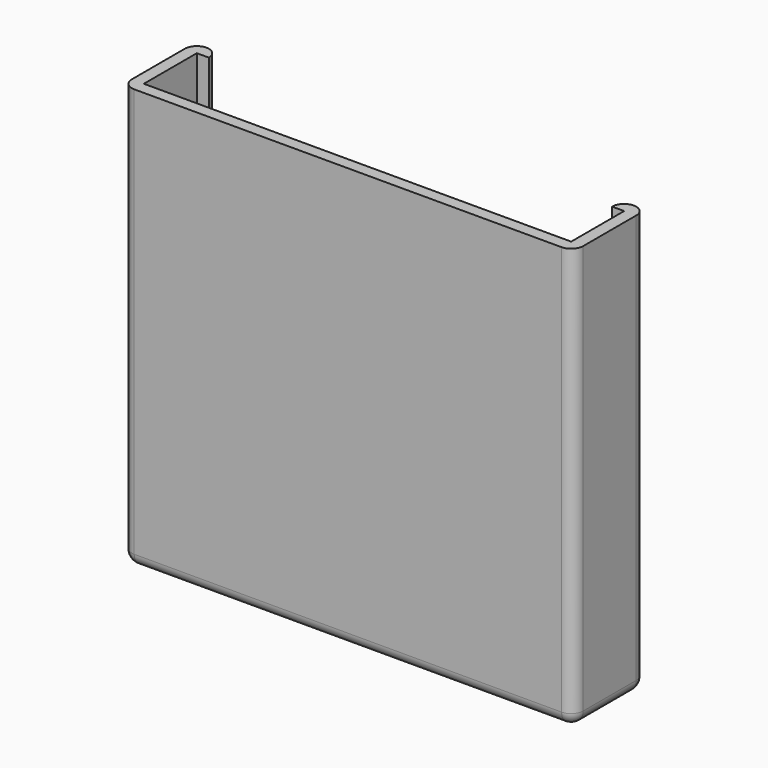
from build123d import *

# Parameters (mm, degrees)
F0_DEPTH     = 70
F1_W         = 75
F1_H         = 15
F4_DEPTH     = 2
F2_T1_DEPTH  = 11
F2_T3_DEPTH  = 73
F2_T5_DEPTH  = 67
F2_T7_DEPTH  = 71
F2_S11_W     = 2.04
F2_S11_H     = 2.04
F2_T12_DEPTH = 2.04
F2_S17_W     = 2.04
F2_S17_H     = 2.04
F2_T18_DEPTH = 2.04
F2_S23_W     = 2.04
F2_S23_H     = 2.04
F2_T24_DEPTH = 2.04
F2_S29_W     = 2.04
F2_S29_H     = 2.04
F2_T30_DEPTH = 2.04
F2_T37_DEPTH = 73
F2_T42_DEPTH = 72
F2_T50_DEPTH = 72
F2_T55_DEPTH = 73
F2_T62_DEPTH = 16
F2_T67_DEPTH = 16


# Not quite as in the source:
# - a fillet or chamfer that OpenCascade refuses, or shapes differently, is made with other operations: its cross-section is extruded or revolved along the edge and cut away or added
# - a feature names something its author has since deleted; it is built from what else it names


with BuildPart() as f0:
    # F3 (on Top) → F0 (new body)
    with BuildSketch(Plane.XY):
        Polygon((-37.5, 15), (-37.5, 0), (37.5, 0), (37.5, 15), (33.5, 15), (33.5, 13), (35.5, 13), (35.5, 2), (-35.5, 2), (-35.5, 13), (-33.5, 13), (-33.5, 15), align=None)
    extrude(amount=F0_DEPTH)

    # F1 (on face) → F4 (join)
    with BuildSketch(Plane(origin=(0, 0, 0), x_dir=(1, 0, 0), z_dir=(0, 0, -1))):
        with Locations((0, -7.5)):
            Rectangle(F1_W, F1_H)
    extrude(amount=-F4_DEPTH)

    # F2: fillet of radius 2 on 13 edges, made by hand

    # F2_s2 → F2_t1 (cut)
    with BuildSketch(Plane.XZ.offset(-13)):
        with BuildLine():
            ThreePointArc((37.5, 2), (36.9142135624, 0.5857864376), (35.5, 0))
            Line((35.5, 0), (37.5, 0))
            Line((37.5, 0), (37.5, 2))
        make_face()
        with BuildLine():
            ThreePointArc((-37.5, 2), (-36.9142135624, 0.5857864376), (-35.5, 0))
            Line((-35.5, 0), (-37.5, 0))
            Line((-37.5, 0), (-37.5, 2))
        make_face()
    extrude(amount=F2_T1_DEPTH, mode=Mode.SUBTRACT)

    # F2_s4 → F2_t3 (cut)
    with BuildSketch(Plane.XY.offset(2)):
        with BuildLine():
            ThreePointArc((-37.5, 2), (-36.9142135624, 0.5857864376), (-35.5, 0))
            Line((-35.5, 0), (-37.5, 0))
            Line((-37.5, 0), (-37.5, 2))
        make_face()
        with BuildLine():
            ThreePointArc((35.5, 0), (36.9142135624, 0.5857864376), (37.5, 2))
            Line((37.5, 2), (37.5, 0))
            Line((37.5, 0), (35.5, 0))
        make_face()
        with BuildLine():
            ThreePointArc((-37.5, 13), (-36.9142135624, 14.4142135624), (-35.5, 15))
            Line((-35.5, 15), (-37.5, 15))
            Line((-37.5, 15), (-37.5, 13))
        make_face()
        with BuildLine():
            ThreePointArc((37.5, 13), (36.9142135624, 14.4142135624), (35.5, 15))
            Line((35.5, 15), (37.5, 15))
            Line((37.5, 15), (37.5, 13))
        make_face()
        with BuildLine():
            ThreePointArc((-33.5, 13), (-34.0857864376, 14.4142135624), (-35.5, 15))
            Line((-35.5, 15), (-33.5, 15))
            Line((-33.5, 15), (-33.5, 13))
        make_face()
        with BuildLine():
            ThreePointArc((33.5, 13), (34.0857864376, 14.4142135624), (35.5, 15))
            Line((35.5, 15), (33.5, 15))
            Line((33.5, 15), (33.5, 13))
        make_face()
    extrude(amount=F2_T3_DEPTH, mode=Mode.SUBTRACT)

    # F2_s6 → F2_t5 (cut)
    with BuildSketch(Plane.YZ.offset(-33.5)):
        with BuildLine():
            ThreePointArc((13, 2), (14.4142135624, 1.4142135624), (15, 0))
            Line((15, 0), (15, 2))
            Line((15, 2), (13, 2))
        make_face()
    extrude(amount=F2_T5_DEPTH, mode=Mode.SUBTRACT)

    # F2_s8 → F2_t7 (cut)
    with BuildSketch(Plane.YZ.offset(-35.5)):
        with BuildLine():
            ThreePointArc((0, 2), (0.5857864376, 0.5857864376), (2, 0))
            Line((2, 0), (0, 0))
            Line((0, 0), (0, 2))
        make_face()
        with BuildLine():
            ThreePointArc((15, 2), (14.4142135624, 0.5857864376), (13, 0))
            Line((13, 0), (15, 0))
            Line((15, 0), (15, 2))
        make_face()
    extrude(amount=F2_T7_DEPTH, mode=Mode.SUBTRACT)


with BuildPart() as f2_tool10:
    # F2_s11 → F2_t12 (new body)
    with BuildSketch(Plane.XZ.offset(-2)):
        with Locations((36.52, 0.98)):
            Rectangle(F2_S11_W, F2_S11_H)
    extrude(amount=F2_T12_DEPTH)

    # F2_s13 → F2_t14 (revolve, cut)
    with BuildSketch(Plane(origin=(35.5, 2, 2), x_dir=(-0.7071067812, 0, 0.7071067812), z_dir=(0.7071067812, 0, 0.7071067812))):
        with BuildLine():
            ThreePointArc((0, -2), (2, 0), (0, 2))
            Line((0, 2), (0, -2))
        make_face()
    revolve(axis=Axis((35.5, 2, 2), (0, -1, 0)), mode=Mode.SUBTRACT)


with BuildPart() as f0_1:
    add(f0.part)

    # F2_t9: cut F2_tool10
    add(f2_tool10.part, mode=Mode.SUBTRACT)


with BuildPart() as f2_tool16:
    # F2_s17 → F2_t18 (new body)
    with BuildSketch(Plane.YZ.offset(35.5)):
        with Locations((14.02, 0.98)):
            Rectangle(F2_S17_W, F2_S17_H)
    extrude(amount=F2_T18_DEPTH)

    # F2_s19 → F2_t20 (revolve, cut)
    with BuildSketch(Plane(origin=(35.5, 13, 2), x_dir=(0, -0.7071067812, 0.7071067812), z_dir=(0, 0.7071067812, 0.7071067812))):
        with BuildLine():
            ThreePointArc((0, -2), (2, 0), (0, 2))
            Line((0, 2), (0, -2))
        make_face()
    revolve(axis=Axis((35.5, 13, 2), (1, 0, 0)), mode=Mode.SUBTRACT)


with BuildPart() as f0_2:
    add(f0_1.part)

    # F2_t15: cut F2_tool16
    add(f2_tool16.part, mode=Mode.SUBTRACT)


with BuildPart() as f2_tool22:
    # F2_s23 → F2_t24 (new body)
    with BuildSketch(Plane.YZ.offset(-35.5)):
        with Locations((14.02, 0.98)):
            Rectangle(F2_S23_W, F2_S23_H)
    extrude(amount=-F2_T24_DEPTH)

    # F2_s25 → F2_t26 (revolve, cut)
    with BuildSketch(Plane(origin=(-35.5, 13, 2), x_dir=(0, -0.7071067812, 0.7071067812), z_dir=(0, -0.7071067812, -0.7071067812))):
        with BuildLine():
            ThreePointArc((0, -2), (2, 0), (0, 2))
            Line((0, 2), (0, -2))
        make_face()
    revolve(axis=Axis((-35.5, 13, 2), (-1, 0, 0)), mode=Mode.SUBTRACT)


with BuildPart() as f0_3:
    add(f0_2.part)

    # F2_t21: cut F2_tool22
    add(f2_tool22.part, mode=Mode.SUBTRACT)


with BuildPart() as f2_tool28:
    # F2_s29 → F2_t30 (new body)
    with BuildSketch(Plane.YZ.offset(-35.5)):
        with Locations((0.98, 0.98)):
            Rectangle(F2_S29_W, F2_S29_H)
    extrude(amount=-F2_T30_DEPTH)

    # F2_s31 → F2_t32 (revolve, cut)
    with BuildSketch(Plane(origin=(-35.5, 2, 2), x_dir=(0, 0.7071067812, 0.7071067812), z_dir=(0, -0.7071067812, 0.7071067812))):
        with BuildLine():
            ThreePointArc((0, -2), (2, 0), (0, 2))
            Line((0, 2), (0, -2))
        make_face()
    revolve(axis=Axis((-35.5, 2, 2), (-1, 0, 0)), mode=Mode.SUBTRACT)


with BuildPart() as f0_4:
    add(f0_3.part)

    # F2_t27: cut F2_tool28
    add(f2_tool28.part, mode=Mode.SUBTRACT)


with BuildPart() as f2_tool35:
    # F2_s36 → F2_t37 (new body)
    with BuildSketch(Plane.XY.offset(-3)):
        with BuildLine():
            ThreePointArc((-33.5, 13), (-34.0857864376, 14.4142135624), (-35.5, 15))
            Line((-35.5, 15), (-33.5, 15))
            Line((-33.5, 15), (-33.5, 13))
        make_face()
    extrude(amount=F2_T37_DEPTH)

    split(bisect_by=Plane.XY.offset(2), keep=Keep.BOTTOM)

    split(bisect_by=Plane.XY, keep=Keep.TOP)


with BuildPart() as f2_tool40:
    # F2_s41 → F2_t42 (new body)
    with BuildSketch(Plane.YZ.offset(-38.5)):
        with BuildLine():
            ThreePointArc((13, 2), (14.4142135624, 1.4142135624), (15, 0))
            Line((15, 0), (15, 2))
            Line((15, 2), (13, 2))
        make_face()
    extrude(amount=F2_T42_DEPTH)

    split(bisect_by=Plane.YZ.offset(-33.5), keep=Keep.BOTTOM)

    split(bisect_by=Plane.YZ.offset(-35.5), keep=Keep.TOP)


with BuildPart() as f2_tool35_1:
    add(f2_tool35.part)

    # F2_t45: intersect F2_tool40
    add(f2_tool40.part, mode=Mode.INTERSECT)


with BuildPart() as f0_5:
    add(f0_4.part)

    # F2_t33: cut F2_tool35
    add(f2_tool35_1.part, mode=Mode.SUBTRACT)


with BuildPart() as f2_tool48:
    # F2_s49 → F2_t50 (new body)
    with BuildSketch(Plane.YZ.offset(-33.5)):
        with BuildLine():
            ThreePointArc((13, 2), (14.4142135624, 1.4142135624), (15, 0))
            Line((15, 0), (15, 2))
            Line((15, 2), (13, 2))
        make_face()
    extrude(amount=F2_T50_DEPTH)

    split(bisect_by=Plane.YZ.offset(35.5), keep=Keep.BOTTOM)

    split(bisect_by=Plane.YZ.offset(33.5), keep=Keep.TOP)


with BuildPart() as f2_tool53:
    # F2_s54 → F2_t55 (new body)
    with BuildSketch(Plane.XY.offset(-3)):
        with BuildLine():
            ThreePointArc((33.5, 13), (34.0857864376, 14.4142135624), (35.5, 15))
            Line((35.5, 15), (33.5, 15))
            Line((33.5, 15), (33.5, 13))
        make_face()
    extrude(amount=F2_T55_DEPTH)

    split(bisect_by=Plane.XY.offset(2), keep=Keep.BOTTOM)

    split(bisect_by=Plane.XY, keep=Keep.TOP)


with BuildPart() as f2_tool48_1:
    add(f2_tool48.part)

    # F2_t58: intersect F2_tool53
    add(f2_tool53.part, mode=Mode.INTERSECT)


with BuildPart() as f0_6:
    add(f0_5.part)

    # F2_t46: cut F2_tool48
    add(f2_tool48_1.part, mode=Mode.SUBTRACT)


with BuildPart() as f2_tool60:
    # F2_s61 → F2_t62 (new body)
    with BuildSketch(Plane.XZ.offset(3)):
        with BuildLine():
            ThreePointArc((35.5, 4), (34.9142135624, 2.5857864376), (33.5, 2))
            Line((33.5, 2), (35.5, 2))
            Line((35.5, 2), (35.5, 4))
        make_face()
    extrude(amount=-F2_T62_DEPTH)

    split(bisect_by=Plane.XZ, keep=Keep.BOTTOM)


with BuildPart() as f0_7:
    add(f0_6.part)

    # F2_t59: union F2_tool60
    add(f2_tool60.part)


with BuildPart() as f2_tool65:
    # F2_s66 → F2_t67 (new body)
    with BuildSketch(Plane.XZ.offset(-13)):
        with BuildLine():
            ThreePointArc((-35.5, 4), (-34.9142135624, 2.5857864376), (-33.5, 2))
            Line((-33.5, 2), (-35.5, 2))
            Line((-35.5, 2), (-35.5, 4))
        make_face()
    extrude(amount=F2_T67_DEPTH)

    split(bisect_by=Plane.XZ, keep=Keep.BOTTOM)


with BuildPart() as f0_8:
    add(f0_7.part)

    # F2_t64: union F2_tool65
    add(f2_tool65.part)


solid = f0_8.part
